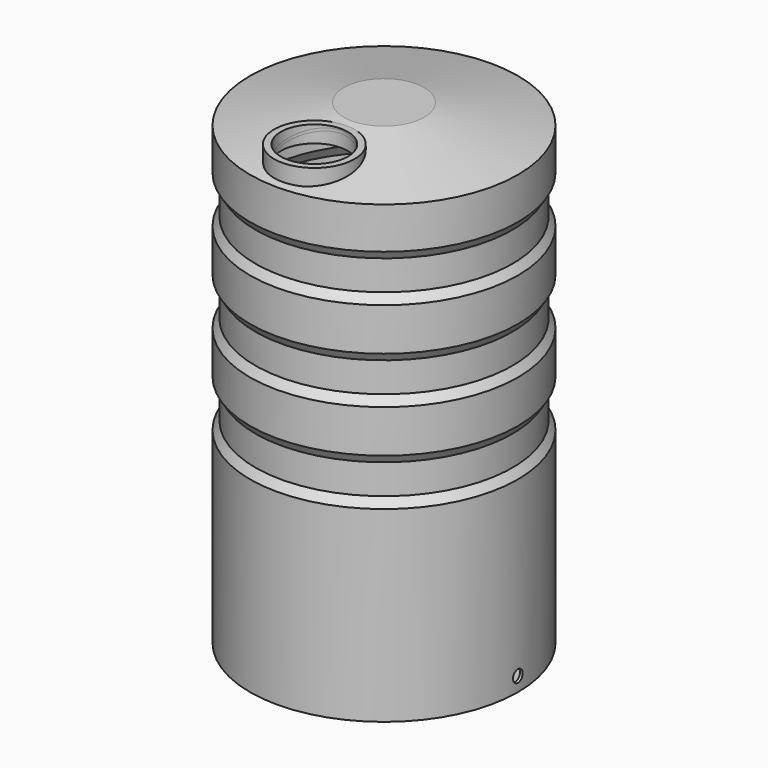
from build123d import *

# Parameters (mm, degrees)
F3_D     = 250
F3_DEPTH = 1000
F3_TIP   = 75.1075773784
F5_D     = 45
F5_DEPTH = 600
F5_TIP   = 13.5193639281
F6_START = -5
F2_R     = 150
F2_R_2   = 125
F6_DEPTH = 62.5


with BuildPart() as f1:
    # F0 (on Front) → F1 (revolve)
    with BuildSketch(Plane.XZ):
        Polygon((-500, -753.3371079093), (0, -753.3371079093), (0, -743.3371079093), (-490, -743.3371079093), (-490, -66.4212658117), (-465, -26.4212658117), (-465, 93.5787341883), (-490, 133.5787341883), (-490, 268.5787341883), (-465, 308.5787341883), (-465, 428.5787341883), (-490, 468.5787341883), (-490, 603.5787341883), (-465, 643.5787341883), (-465, 763.5787341883), (-490, 803.5787341883), (-490, 938.5787341883), (-148.9405964557, 1011.6628920907), (0, 1011.6628920907), (0, 1021.6628920907), (-150, 1021.6628920907), (-500, 946.6628920907), (-500, 791.2767907922), (-480, 759.2767907922), (-480, 647.8806775845), (-500, 615.8806775845), (-500, 456.2767907922), (-480, 424.2767907922), (-480, 312.8806775845), (-500, 280.8806775845), (-500, 121.2767907922), (-480, 89.2767907922), (-480, -22.1193224155), (-500, -54.1193224155), align=None)
    revolve(axis=Axis((0, 0, 139.1628920907), (0, 0, -1)))

    # F3
    with Locations(Plane.XY.offset(1021.6628920907)):
        with Locations((0, -325)):
            Hole(F3_D / 2, depth=F3_DEPTH)
            with Locations((0, 0, -(F3_DEPTH + F3_TIP / 2))):  # 118° drill point
                Cone(0, F3_D / 2, F3_TIP, mode=Mode.SUBTRACT)

    # F5 (one way)
    with BuildSketch(Plane(origin=(0, 0, 0), x_dir=(0, 1, 0), z_dir=(-1, 0, 0))):
        with Locations((0, 700)):
            Circle(F5_D / 2)
    extrude(amount=-F5_DEPTH, mode=Mode.SUBTRACT)
    with Locations(Plane(origin=(0, 0, 0), x_dir=(0, 1, 0), z_dir=(-1, 0, 0))):
        with Locations((0, 700)):
            with Locations((0, 0, -(F5_DEPTH + F5_TIP / 2))):  # 118° drill point
                Cone(0, F5_D / 2, F5_TIP, mode=Mode.SUBTRACT)

    # F2 (on face) → F6 (join)
    with BuildSketch(Plane.XY.offset(1021.6628920907).offset(F6_START)):
        with Locations((0, -325)):
            Circle(F2_R)
        with Locations((0, -325)):
            Circle(F2_R_2, mode=Mode.SUBTRACT)
    extrude(amount=-F6_DEPTH)


solid = f1.part
